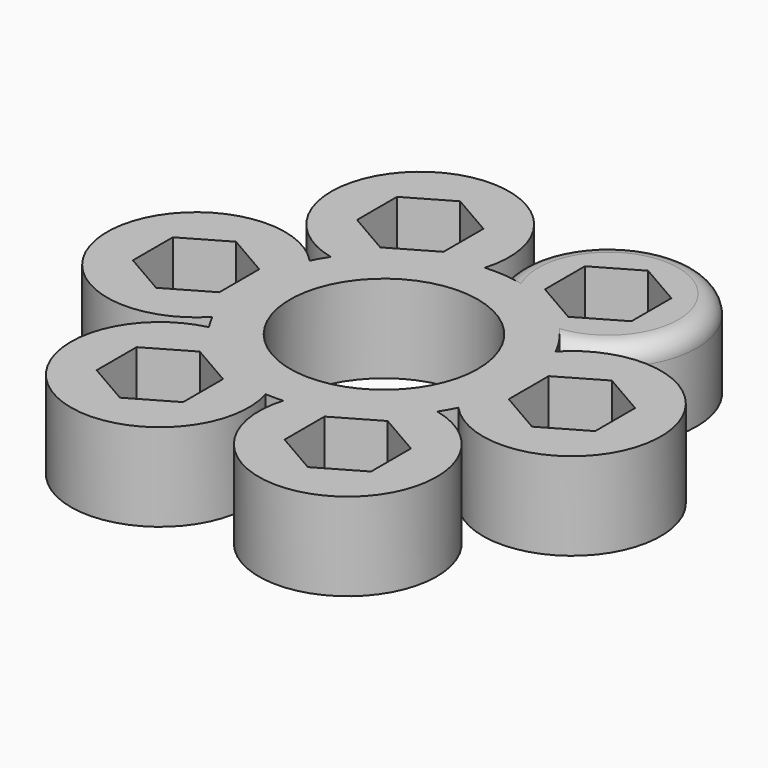
from build123d import *

# Parameters (mm, degrees)
F0_R        = 7.5
F1_DEPTH    = 7
F2_T4_ANGLE = 334.5116796515
F2_S5_R     = 10.95
F2_T6_DEPTH = 12


# Not quite as in the source:
# - a fillet or chamfer that OpenCascade refuses, or shapes differently, is made with other operations: its cross-section is extruded or revolved along the edge and cut away or added


with BuildPart() as f1:
    # F0 (on Top) → F1 (new body)
    with BuildSketch(Plane.XY):
        with BuildLine():
            ThreePointArc((-9.8156361058, 4.8534305226), (-22.1016488807, 0), (-9.8156361058, -4.8534305226))
            ThreePointArc((-9.8156361058, -4.8534305226), (-9.4829781714, -5.475), (-9.111012181, -6.0738749607))
            ThreePointArc((-9.111012181, -6.0738749607), (-11.0508244404, -19.1405893962), (-0.7046239248, -10.9273054833))
            ThreePointArc((-0.7046239248, -10.9273054833), (0, -10.95), (0.7046239248, -10.9273054833))
            ThreePointArc((0.7046239248, -10.9273054833), (11.0508244404, -19.1405893962), (9.111012181, -6.0738749607))
            ThreePointArc((9.111012181, -6.0738749607), (9.4829781714, -5.475), (9.8156361058, -4.8534305226))
            ThreePointArc((9.8156361058, -4.8534305226), (22.1016488807, 0), (9.8156361058, 4.8534305226))
            ThreePointArc((9.8156361058, 4.8534305226), (9.4829781714, 5.475), (9.111012181, 6.0738749607))
            ThreePointArc((9.111012181, 6.0738749607), (11.0508244404, 19.1405893962), (0.7046239248, 10.9273054833))
            ThreePointArc((0.7046239248, 10.9273054833), (0, 10.95), (-0.7046239248, 10.9273054833))
            ThreePointArc((-0.7046239248, 10.9273054833), (-11.0508244404, 19.1405893962), (-9.111012181, 6.0738749607))
            ThreePointArc((-9.111012181, 6.0738749607), (-9.4829781714, 5.475), (-9.8156361058, 4.8534305226))
        make_face()
        Polygon((-4.05, -14.9822394855), (-7.5, -16.9740979142), (-10.95, -14.9822394855), (-10.95, -10.9985226281), (-7.5, -9.0066641994), (-4.05, -10.9985226281), align=None, mode=Mode.SUBTRACT)
        Polygon((10.95, -10.9985226281), (10.95, -14.9822394855), (7.5, -16.9740979142), (4.05, -14.9822394855), (4.05, -10.9985226281), (7.5, -9.0066641994), align=None, mode=Mode.SUBTRACT)
        Polygon((-15, 3.9837168574), (-11.55, 1.9918584287), (-11.55, -1.9918584287), (-15, -3.9837168574), (-18.45, -1.9918584287), (-18.45, 1.9918584287), align=None, mode=Mode.SUBTRACT)
        Polygon((-10.95, 10.9985226281), (-10.95, 14.9822394855), (-7.5, 16.9740979142), (-4.05, 14.9822394855), (-4.05, 10.9985226281), (-7.5, 9.0066641994), align=None, mode=Mode.SUBTRACT)
        Circle(F0_R, mode=Mode.SUBTRACT)
        Polygon((15, 3.9837168574), (18.45, 1.9918584287), (18.45, -1.9918584287), (15, -3.9837168574), (11.55, -1.9918584287), (11.55, 1.9918584287), align=None, mode=Mode.SUBTRACT)
        Polygon((4.05, 14.9822394855), (7.5, 16.9740979142), (10.95, 14.9822394855), (10.95, 10.9985226281), (7.5, 9.0066641994), (4.05, 10.9985226281), align=None, mode=Mode.SUBTRACT)
    extrude(amount=F1_DEPTH)

    # F2: fillet of radius 1.5 on 1 edges, made by hand


with BuildPart() as f2_tool2:
    # F2_s3 → F2_t4 (revolve)
    with BuildSketch(Plane(origin=(3.1600326445, -0.9815693661, 0), x_dir=(0, 0, 1), z_dir=(-0.9549897147, 0.2966389131, 0))):
        with BuildLine():
            ThreePointArc((5.5, 7.528823267), (6.5606601718, 7.9681630952), (7, 9.028823267))
            Line((7, 9.028823267), (7, 7.528823267))
            Line((7, 7.528823267), (5.5, 7.528823267))
        make_face()
    revolve(axis=Axis((7.5, 12.9903810568, 7), (0, 0, 1)), revolution_arc=F2_T4_ANGLE)

    # F2_s5 → F2_t6 (cut, symmetric)
    with BuildSketch(Plane.XY.offset(6.2)):
        Circle(F2_S5_R)
    extrude(amount=F2_T6_DEPTH, both=True, mode=Mode.SUBTRACT)


with BuildPart() as f1_1:
    add(f1.part)

    # F2_t1: cut F2_tool2
    add(f2_tool2.part, mode=Mode.SUBTRACT)


solid = f1_1.part
